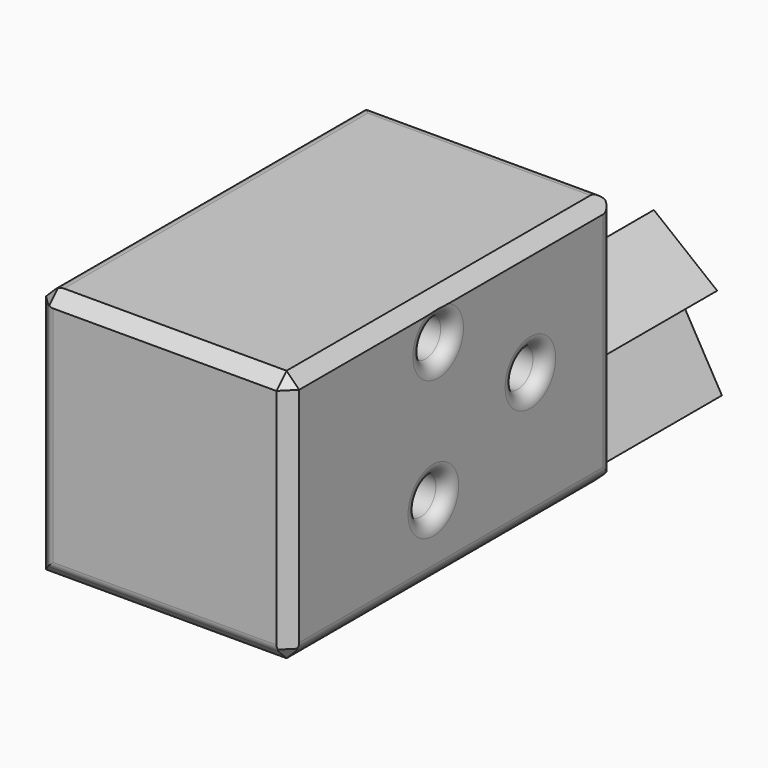
from build123d import *

# Parameters (mm, degrees)
F0_W        = 127
F0_H        = 127
F1_DEPTH    = 203.2
F3_D        = 19.05
F4_SIZE     = 6.35
F5_T1_DEPTH = 210.0012806053
F5_T3_DEPTH = 146.05
F5_T5_DEPTH = 146.05
F6_R        = 5.08
F7_R        = 5.08
F9_DEPTH    = 76.2


# Not quite as in the source:
# - a fillet or chamfer that OpenCascade refuses, or shapes differently, is made with other operations: its cross-section is extruded or revolved along the edge and cut away or added


with BuildPart() as f1:
    # F0 (on Front) → F1 (new body)
    with BuildSketch(Plane.XZ):
        with Locations((63.5, 63.5)):
            Rectangle(F0_W, F0_H)
    extrude(amount=F1_DEPTH)

    # F3 (through all)
    with Locations(Plane.YZ.offset(127)):
        with Locations((-109.707146883, 106.2569767237), (-51.8769121036, 69.3713248935), (-112.7359410134, 37.7316983828)):
            Hole(F3_D / 2)

    # F4
    f4_edges = [f1.edges().sort_by_distance(p)[0] for p in [
        (63.5, -203.2, 127),
        (0, -203.2, 63.5),
        (127, -203.2, 63.5),
        (63.5, -203.2, 0),
        (127, -101.6, 0),
        (127, -101.6, 127),
        (0, -101.6, 127),
    ]]
    chamfer(f4_edges, length=F4_SIZE)

    # F5: fillet of radius 6.35 on 7 edges, made by hand

    # F5_s2 → F5_t1 (cut)
    with BuildSketch(Plane.XZ.offset(-6.5756403027)):
        with BuildLine():
            ThreePointArc((4.4901280605, 125.1401280605), (6.5502163256, 126.5166350314), (8.9802561211, 127))
            Line((8.9802561211, 127), (6.35, 127))
            Line((6.35, 127), (4.4901280605, 125.1401280605))
        make_face()
        with BuildLine():
            ThreePointArc((125.1401280605, 4.4901280605), (126.5166350314, 6.5502163256), (127, 8.9802561211))
            Line((127, 8.9802561211), (127, 6.35))
            Line((127, 6.35), (125.1401280605, 4.4901280605))
        make_face()
    extrude(amount=F5_T1_DEPTH, mode=Mode.SUBTRACT)

    # F5_s4 → F5_t3 (cut)
    with BuildSketch(Plane.YZ.offset(-9.525)):
        with BuildLine():
            ThreePointArc((0, 120.65), (-1.8598719395, 125.1401280605), (-6.35, 127))
            Line((-6.35, 127), (0, 127))
            Line((0, 127), (0, 120.65))
        make_face()
    extrude(amount=F5_T3_DEPTH, mode=Mode.SUBTRACT)

    # F5_s6 → F5_t5 (cut)
    with BuildSketch(Plane.XY.offset(-9.525)):
        with BuildLine():
            ThreePointArc((120.65, 0), (125.1401280605, -1.8598719395), (127, -6.35))
            Line((127, -6.35), (127, 0))
            Line((127, 0), (120.65, 0))
        make_face()
    extrude(amount=F5_T5_DEPTH, mode=Mode.SUBTRACT)

    # F5_s7 → F5_t8 (revolve, cut)
    with BuildSketch(Plane.XY.offset(106.2569767237)):
        with BuildLine():
            ThreePointArc((120.65, -100.182146883), (125.1401280605, -98.3222749435), (127, -93.832146883))
            Line((127, -93.832146883), (127, -100.182146883))
            Line((127, -100.182146883), (120.65, -100.182146883))
        make_face()
    revolve(axis=Axis((127, -109.707146883, 106.2569767237), (1, 0, 0)), mode=Mode.SUBTRACT)

    # F5_s9 → F5_t10 (revolve, cut)
    with BuildSketch(Plane.XY.offset(37.7316983828)):
        with BuildLine():
            ThreePointArc((120.65, -103.2109410134), (125.1401280605, -101.3510690739), (127, -96.8609410134))
            Line((127, -96.8609410134), (127, -103.2109410134))
            Line((127, -103.2109410134), (120.65, -103.2109410134))
        make_face()
    revolve(axis=Axis((127, -112.7359410134, 37.7316983828), (1, 0, 0)), mode=Mode.SUBTRACT)

    # F5_s11 → F5_t12 (revolve, cut)
    with BuildSketch(Plane.XY.offset(69.3713248935)):
        with BuildLine():
            ThreePointArc((120.65, -42.3519121036), (125.1401280605, -40.4920401641), (127, -36.0019121036))
            Line((127, -36.0019121036), (127, -42.3519121036))
            Line((127, -42.3519121036), (120.65, -42.3519121036))
        make_face()
    revolve(axis=Axis((127, -51.8769121036, 69.3713248935), (1, 0, 0)), mode=Mode.SUBTRACT)

    # F6
    f6_edges = [f1.edges().sort_by_distance(p)[0] for p in [
        (6.35, -203.2, 63.5),
        (63.5, -203.2, 6.35),
    ]]
    fillet(f6_edges, radius=F6_R)

    # F7
    f7_edges = [f1.edges().sort_by_distance(p)[0] for p in [
        (60.325, 0, 0),
        (0, 0, 60.325),
    ]]
    fillet(f7_edges, radius=F7_R)

    # F8 (on face) → F9 (join)
    with BuildSketch(Plane(origin=(0, 0, 0), x_dir=(-1, 0, 0), z_dir=(0, 1, 0))):
        Polygon((-100.4286549397, 40.3320468052), (-120.65, 5.08), (-54.4255593013, 5.08), (-54.4255593013, 9.1751408411), (-75.2091502909, 31.4702691336), (-64.1732869808, 55.1769325335), (-86.5088332529, 75.9170813451), (-118.2750036349, 50.5691027419), align=None)
    extrude(amount=F9_DEPTH)


solid = f1.part
